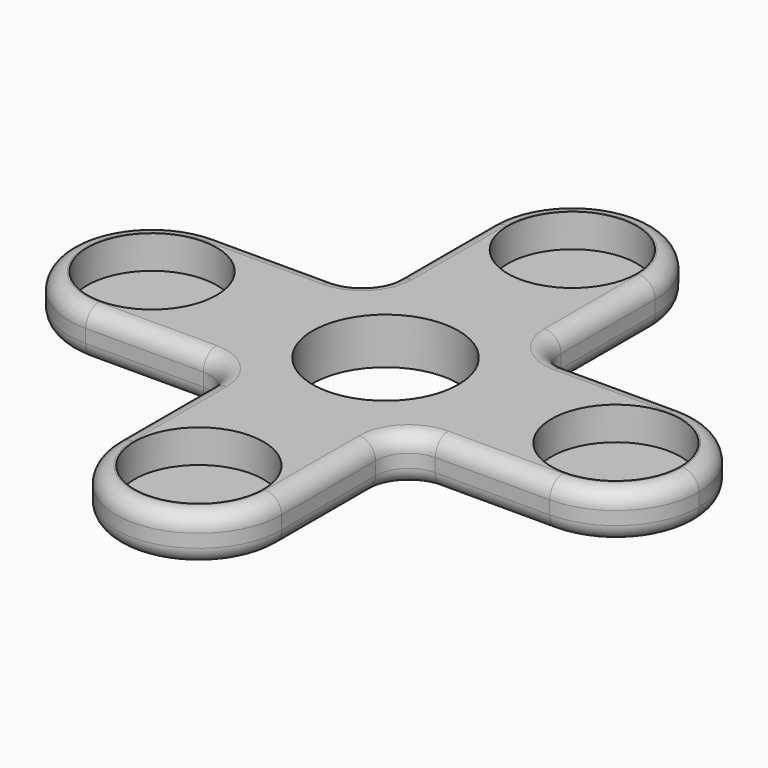
from build123d import *

# Parameters (mm, degrees)
F0_R     = 9.75
F0_R_2   = 11
F1_DEPTH = 7
F2_R     = 2.5
F3_DEPTH = 2


# Not quite as in the source:
# - ends of sketch curves that miss each other by under 0.0002 mm in the source are joined


with BuildPart() as f1:
    # F0 (on Top) → F1 (new body)
    with BuildSketch(Plane.XY):
        with BuildLine():
            ThreePointArc((-124.122170751, 0), (-111.622170751, -12.5), (-99.122170751, 0))
            ThreePointArc((-99.122170751, 0), (-111.622170751, 12.5), (-124.122170751, 0))
        make_face()
        with Locations((-111.6057372503, 0)):
            Circle(F0_R, mode=Mode.SUBTRACT)
        with BuildLine():
            ThreePointArc((-124.122170751, 70.4979732546), (-111.622170751, 57.9979732546), (-99.122170751, 70.4979732546))
            ThreePointArc((-99.122170751, 70.4979732546), (-111.622170751, 82.9979732546), (-124.122170751, 70.4979732546))
        make_face()
        with Locations((-111.622170751, 70.4979732546)):
            Circle(F0_R, mode=Mode.SUBTRACT)
        with BuildLine():
            ThreePointArc((-64.3390744925, 35.2479732546), (-68.0002397276, 44.0868080194), (-76.8390744925, 47.7479732546))
            ThreePointArc((-76.8390744925, 47.7479732546), (-89.3390744925, 35.2479732546), (-76.8390744925, 22.7479732546))
            ThreePointArc((-76.8390744925, 22.7479732546), (-68.0002397276, 26.4091384898), (-64.3390744925, 35.2479732546))
        make_face()
        with Locations((-76.8390744925, 35.2479732546)):
            Circle(F0_R, mode=Mode.SUBTRACT)
        with BuildLine():
            Line((-99.122170751, 52.7479732546), (-99.122170751, 70.4979732546))
            ThreePointArc((-99.122170751, 70.4979732546), (-111.622170751, 57.9979732546), (-124.122170751, 70.4979732546))
            Line((-124.122170751, 70.4979732546), (-124.122170751, 52.7479732546))
            ThreePointArc((-124.122170751, 52.7479732546), (-125.5866368451, 49.2124393487), (-129.122170751, 47.7479732546))
            Line((-129.122170751, 47.7479732546), (-146.872170751, 47.7479732546))
            ThreePointArc((-146.872170751, 47.7479732546), (-138.0333359862, 44.0868088626), (-134.372170751, 35.2479740977))
            ThreePointArc((-134.372170751, 35.2479740977), (-138.0333359862, 26.4091393329), (-146.872170751, 22.7479740977))
            Line((-146.872170751, 22.7479740977), (-129.122170751, 22.7479740977))
            ThreePointArc((-129.122170751, 22.7479740977), (-125.5866368451, 21.2835080037), (-124.122170751, 17.7479740977))
            Line((-124.122170751, 17.7479740977), (-124.122170751, 0))
            ThreePointArc((-124.122170751, 0), (-111.622170751, 12.5), (-99.122170751, 0))
            Line((-99.122170751, 0), (-99.122170751, 17.7479740977))
            ThreePointArc((-99.122170751, 17.7479740977), (-97.6577046569, 21.2835080037), (-94.122170751, 22.7479740977))
            Line((-94.122170751, 22.7479740977), (-76.8390744925, 22.7479740977))
            ThreePointArc((-76.8390744925, 22.7479740977), (-89.3390744925, 35.2479732546), (-76.8390744925, 47.7479732546))
            Line((-76.8390744925, 47.7479732546), (-94.122170751, 47.7479732546))
            ThreePointArc((-94.122170751, 47.7479732546), (-97.6577046569, 49.2124393487), (-99.122170751, 52.7479732546))
        make_face()
        with Locations((-111.622170751, 35.2479732546)):
            Circle(F0_R_2, mode=Mode.SUBTRACT)
        with BuildLine():
            ThreePointArc((-134.372170751, 35.2479740977), (-138.0333359862, 44.0868088626), (-146.872170751, 47.7479740977))
            ThreePointArc((-146.872170751, 47.7479740977), (-159.372170751, 35.2479740977), (-146.872170751, 22.7479740977))
            ThreePointArc((-146.872170751, 22.7479740977), (-138.0333359862, 26.4091393329), (-134.372170751, 35.2479740977))
        make_face()
        with Locations((-146.872170751, 35.2479732546)):
            Circle(F0_R, mode=Mode.SUBTRACT)
    extrude(amount=F1_DEPTH)

    # F2
    f2_edges = [f1.edges().sort_by_distance(p)[0] for p in [
        (-124.122171, 61.622973, 7),
        (-125.586637, 49.212439, 7),
        (-137.997171, 22.747974, 0),
        (-125.586637, 21.283508, 0),
        (-124.122171, 8.873987, 0),
        (-111.622171, -12.5, 7),
        (-99.122171, 8.873987, 0),
        (-111.622171, -12.5, 0),
        (-111.622171, 82.997973, 7),
        (-99.122171, 61.622973, 7),
        (-97.657705, 49.212439, 7),
        (-85.480623, 47.747973, 7),
        (-64.339074, 35.247973, 7),
        (-85.480623, 22.747974, 7),
        (-97.657705, 21.283508, 7),
        (-99.122171, 8.873987, 7),
        (-159.372171, 35.247974, 7),
        (-137.997171, 47.747973, 7),
        (-124.122171, 8.873987, 7),
        (-125.586637, 21.283508, 7),
        (-137.997171, 22.747974, 7),
        (-97.657705, 21.283508, 0),
        (-85.480623, 22.747974, 0),
        (-64.339074, 35.247973, 0),
        (-85.480623, 47.747973, 0),
        (-111.622171, 82.997973, 0),
        (-97.657705, 49.212439, 0),
        (-99.122171, 61.622973, 0),
        (-124.122171, 61.622973, 0),
        (-125.586637, 49.212439, 0),
        (-137.997171, 47.747973, 0),
        (-159.372171, 35.247974, 0),
    ]]
    fillet(f2_edges, radius=F2_R)

    # F0 (on Top) → F3 (join)
    with BuildSketch(Plane.XY):
        with Locations((-76.8390744925, 35.2479732546)):
            Circle(F0_R)
        with Locations((-111.622170751, 70.4979732546)):
            Circle(F0_R)
        with Locations((-146.872170751, 35.2479732546)):
            Circle(F0_R)
        with Locations((-111.6057372503, 0)):
            Circle(F0_R)
    extrude(amount=F3_DEPTH)


solid = f1.part
